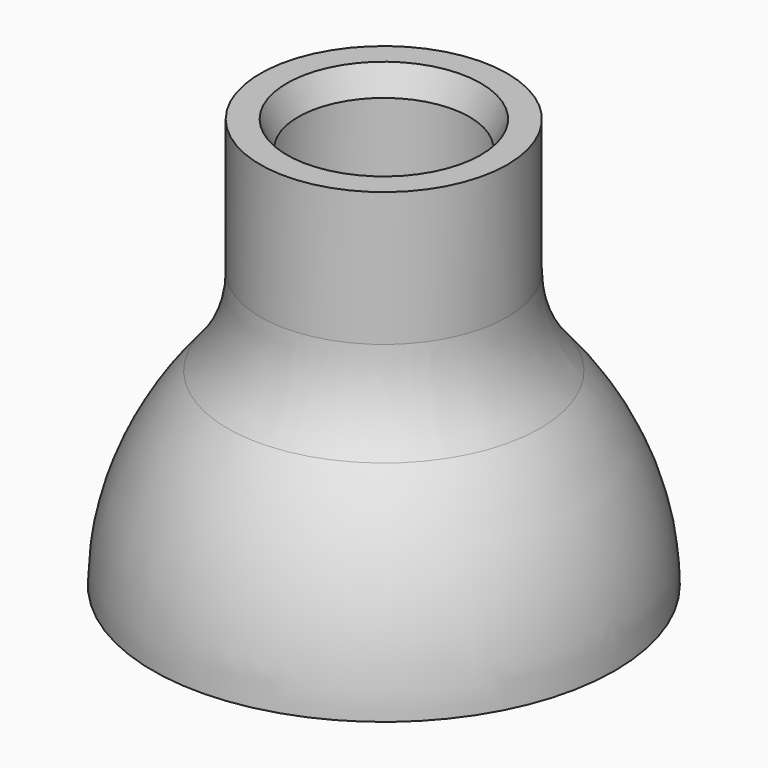
from build123d import *


# Not quite as in the source:
# - ends of sketch curves that miss each other by under 0.0002 mm in the source are joined
# - the dataset's text gives a spline's control points without its knots; the knots are read off the source's solid


with BuildPart() as f1:
    # F0 (on Front) → F1 (revolve)
    with BuildSketch(Plane.XZ):
        Polygon((9.7069498152, 15.0171099231), (11, 15.0171099231), (11, 17.9548243945), align=None)
        with BuildLine():
            Line((11, 15.0171099231), (11, 10.5107510462))
            Line((11, 10.5107510462), (11, -4.9711427956))
            add(Edge.make_bspline(
                [(11, -4.9711427956), (16.2437419004, -8.8163125959), (23.19943312, -17.5511940928), (23.1994349799, -28.5690823316)],
                knots=[0, 0, 0, 0, 26.5648068726, 26.5648068726, 26.5648068726, 26.5648068726], degree=3))
            Line((23.1994349799, -28.5690823316), (26.1994349799, -28.5690823316))
            add(Edge.make_bspline(
                [(17.7265217002, -7.1481812805), (19.1095590047, -8.7235328339), (21.9155043848, -12.5059639132), (25.2274131623, -19.6838085881), (26.1994344616, -25.4989553681), (26.1994349799, -28.5690823316)],
                knots=[0.2712350474, 0.2712350474, 0.2712350474, 0.2712350474, 0.5, 0.75, 1, 1, 1, 1], degree=3))
            ThreePointArc((17.7265217002, -7.1481812805), (14.962499563, -2.5400303169), (14, 2.7466114794))
            Line((14, 2.7466114794), (14, 17.9548243945))
            Line((14, 17.9548243945), (11, 17.9548243945))
            Line((11, 17.9548243945), (11, 15.0171099231))
        make_face()
    revolve(axis=Axis((0, 0, 14.5892715082), (0, 0, 1)))


solid = f1.part
